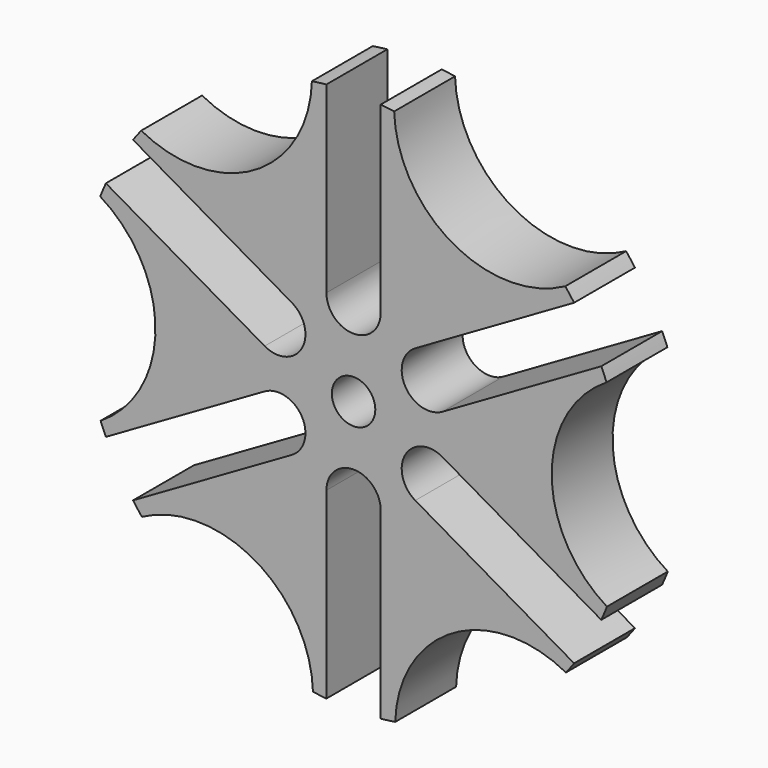
from build123d import *

# Parameters (mm, degrees)
F0_R            = 25
F1_DEPTH        = 7
F3_DEPTH        = 13.3
F3_COPIES_COUNT = 6
F4_R            = 2
F5_DEPTH        = 25


# Not quite as in the source:
# - a pattern or mirror of a feature is missing from the dataset's text; its kind, count and spacing are read off the source's solid


with BuildPart() as f1:
    # F0 (on Front) → F1 (new body)
    with BuildSketch(Plane.XZ):
        Circle(F0_R)
    extrude(amount=F1_DEPTH)

    # F2 (on face) → F3 (cut)
    with BuildSketch(Plane.XZ.offset(7)):
        with BuildLine():
            ThreePointArc((-19.5394295308, 15.5952138046), (-12.5429522443, 21.6257797315), (-3.8342431732, 24.704221892))
            ThreePointArc((-3.8342431732, 24.704221892), (-3.8311679177, 24.8520967356), (-3.8301427668, 25))
            ThreePointArc((-3.8301427668, 25), (-19.9806869892, 34.1546667609), (-19.5394295308, 15.5952138046))
        make_face()
        with BuildLine():
            ThreePointArc((-19.5394295308, 15.5952138046), (-9.1467396108, 15.7702407083), (-3.8342431732, 24.704221892))
            ThreePointArc((-3.8342431732, 24.704221892), (-12.5429522443, 21.6257797315), (-19.5394295308, 15.5952138046))
        make_face()
        with BuildLine():
            ThreePointArc((2.4968730444, 24.875), (2.4992181388, 24.9374804474), (2.5, 25))
            ThreePointArc((2.5, 25), (0, 27.5), (-2.5, 25))
            ThreePointArc((-2.5, 25), (-2.4992181388, 24.9374804474), (-2.4968730444, 24.875))
            ThreePointArc((-2.4968730444, 24.875), (0, 25), (2.4968730444, 24.875))
        make_face()
        with BuildLine():
            ThreePointArc((-2.4968730444, 24.875), (0, 22.5), (2.4968730444, 24.875))
            ThreePointArc((2.4968730444, 24.875), (0, 25), (-2.4968730444, 24.875))
        make_face()
        with BuildLine():
            ThreePointArc((2.5, 24.8746859277), (2.4984365271, 24.874843013), (2.4968730444, 24.875))
            ThreePointArc((2.4968730444, 24.875), (0, 22.5), (-2.4968730444, 24.875))
            ThreePointArc((-2.4968730444, 24.875), (-2.4984365271, 24.874843013), (-2.5, 24.8746859277))
            Line((-2.5, 24.8746859277), (-2.5, 8))
            ThreePointArc((-2.5, 8), (0, 10.5), (2.5, 8))
            Line((2.5, 8), (2.5, 24.8746859277))
        make_face()
        with BuildLine():
            ThreePointArc((-2.5, 8), (0, 5.5), (2.5, 8))
            ThreePointArc((2.5, 8), (0, 10.5), (-2.5, 8))
        make_face()
    f3 = extrude(amount=-F3_DEPTH, mode=Mode.SUBTRACT)

    # F3_copies: F3 ×6 about axis
    f3_copies_axis = Axis((0, 0, 0), (0, 1, 0))
    for i in range(1, F3_COPIES_COUNT):
        add(f3.rotate(f3_copies_axis, i * 360 / F3_COPIES_COUNT), mode=Mode.SUBTRACT)

    # F4 (on face) → F5 (cut)
    with BuildSketch(Plane.XZ.offset(7)):
        Circle(F4_R)
    extrude(amount=-F5_DEPTH, mode=Mode.SUBTRACT)


solid = f1.part
